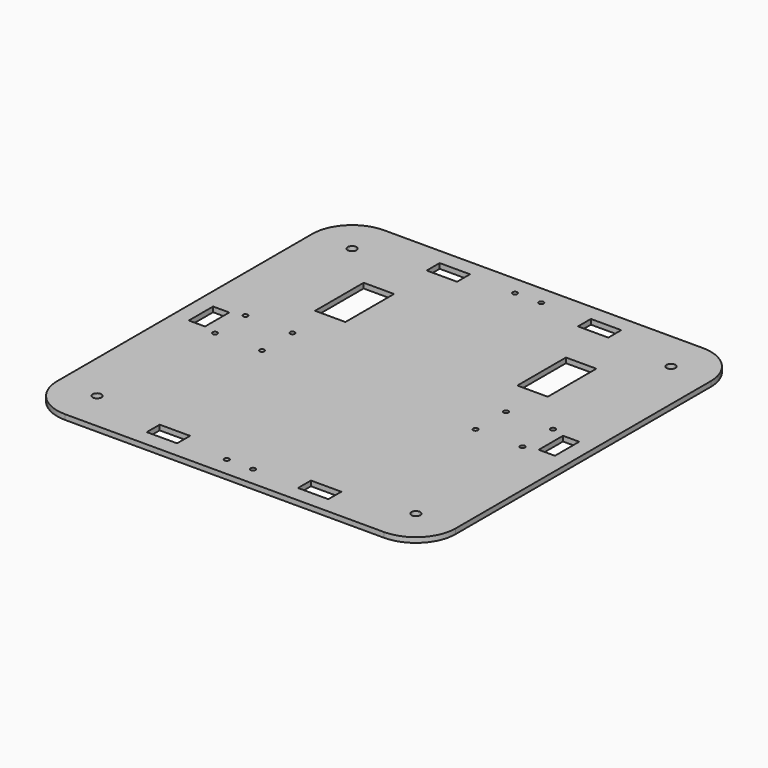
from build123d import *

# Parameters (mm, degrees)
F0_R     = 2.7608867496
F0_W     = 19.05
F0_H     = 10.16
F0_R_2   = 1.5
F0_W_2   = 10.16
F0_H_2   = 19.05
F0_H_3   = 38.1
F1_DEPTH = 3.175


# Not quite as in the source:
# - a length typed as a fraction of an inch, garbled in the dataset ("3 / 203.2 mm" for 3/8 in), is restored


with BuildPart() as f1:
    # F0 (on Top) → F1 (new body)
    with BuildSketch(Plane.XY):
        with BuildLine():
            Line((100, 125), (-100, 125))
            ThreePointArc((-100, 125), (-117.6776695297, 117.6776695297), (-125, 100))
            Line((-125, 100), (-125, -100))
            ThreePointArc((-125, -100), (-117.6776695297, -117.6776695297), (-100, -125))
            Line((-100, -125), (100, -125))
            ThreePointArc((100, -125), (117.6776695297, -117.6776695297), (125, -100))
            Line((125, -100), (125, 100))
            ThreePointArc((125, 100), (117.6776695297, 117.6776695297), (100, 125))
        make_face()
        with Locations((-100, -100)):
            Circle(F0_R, mode=Mode.SUBTRACT)
        with Locations((-47.4411445916, -109.76)):
            Rectangle(F0_W, F0_H, mode=Mode.SUBTRACT)
        with Locations((-8.23, -113)):
            Circle(F0_R_2, mode=Mode.SUBTRACT)
        with Locations((-96.4635497928, -11.935)):
            Circle(F0_R_2, mode=Mode.SUBTRACT)
        with Locations((-66.9635497928, -11.935)):
            Circle(F0_R_2, mode=Mode.SUBTRACT)
        with Locations((8.23, -113)):
            Circle(F0_R_2, mode=Mode.SUBTRACT)
        with Locations((47.4411445916, -109.76)):
            Rectangle(F0_W, F0_H, mode=Mode.SUBTRACT)
        with Locations((100, -100)):
            Circle(F0_R, mode=Mode.SUBTRACT)
        with Locations((66.9635497928, -11.935)):
            Circle(F0_R_2, mode=Mode.SUBTRACT)
        with Locations((96.4635497928, -11.935)):
            Circle(F0_R_2, mode=Mode.SUBTRACT)
        with Locations((-109.76, 0)):
            Rectangle(F0_W_2, F0_H_2, mode=Mode.SUBTRACT)
        with Locations((-96.4635497928, 11.935)):
            Circle(F0_R_2, mode=Mode.SUBTRACT)
        with Locations((-66.9635497928, 11.935)):
            Circle(F0_R_2, mode=Mode.SUBTRACT)
        with Locations((-63.4532595247, 56.2142550719)):
            Rectangle(F0_W, F0_H_3, mode=Mode.SUBTRACT)
        with Locations((-100, 100)):
            Circle(F0_R, mode=Mode.SUBTRACT)
        with Locations((-47.4411445916, 109.76)):
            Rectangle(F0_W, F0_H, mode=Mode.SUBTRACT)
        with Locations((-8.23, 113)):
            Circle(F0_R_2, mode=Mode.SUBTRACT)
        with Locations((66.9635497928, 11.935)):
            Circle(F0_R_2, mode=Mode.SUBTRACT)
        with Locations((96.4635497928, 11.935)):
            Circle(F0_R_2, mode=Mode.SUBTRACT)
        with Locations((109.76, 0)):
            Rectangle(F0_W_2, F0_H_2, mode=Mode.SUBTRACT)
        with Locations((63.4532595247, 56.2142550719)):
            Rectangle(F0_W, F0_H_3, mode=Mode.SUBTRACT)
        with Locations((8.23, 113)):
            Circle(F0_R_2, mode=Mode.SUBTRACT)
        with Locations((47.4411445916, 109.76)):
            Rectangle(F0_W, F0_H, mode=Mode.SUBTRACT)
        with Locations((100, 100)):
            Circle(F0_R, mode=Mode.SUBTRACT)
    extrude(amount=F1_DEPTH)


solid = f1.part
